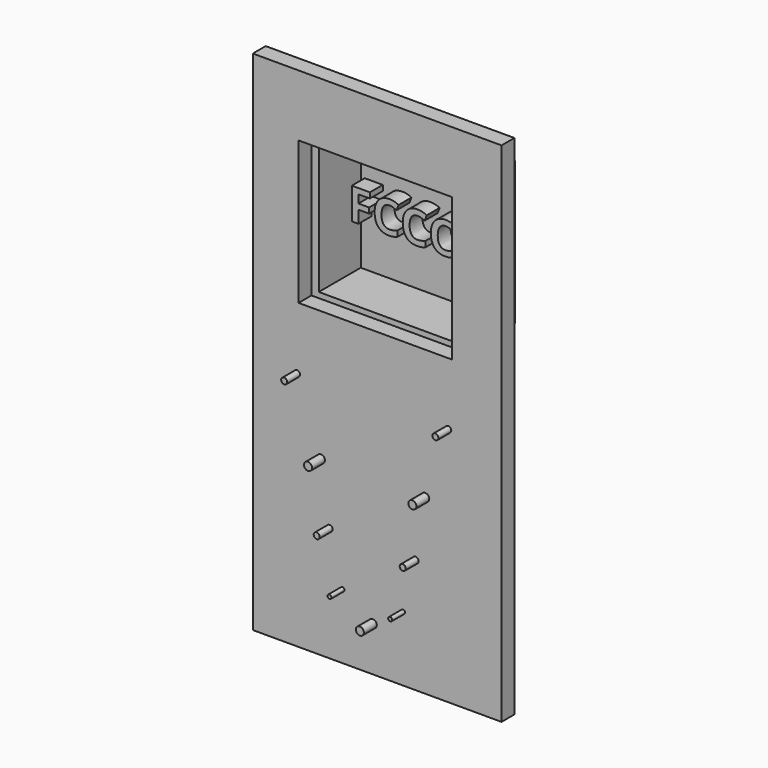
from build123d import *

# Parameters (mm, degrees)
F0_W         = 392.2961652279
F0_H         = 800.5814924836
F0_W_2       = 242.1113476157
F0_H_2       = 225.6477475166
F1_DEPTH     = 25.4
F2_R         = 6.35
F2_R_2       = 3.175
F2_R_3       = 4.7625
F3_DEPTH     = 25.4
F4_W         = 242.1113476157
F4_H         = 225.6477475166
F5_DEPTH     = 99.06
F6_W         = 223.6813679338
F6_H         = 208.9384496212
F7_DEPTH     = 82.804
F8_TEXT_SIZE = 69.5675359498
F9_DEPTH     = 25.4


# Not quite as in the source:
# - Text() gives the source's letters only with a copy of the font that has no kerning and outlines rounded to 1/6400 em; it was checked with that copy


with BuildPart() as f1:
    # F0 (on Front) → F1 (new body)
    with BuildSketch(Plane.XZ):
        with Locations((6.9621950388, 280.5182151496)):
            Rectangle(F0_W, F0_H)
        with Locations((4.0568597615, 470.8177149296)):
            Rectangle(F0_W_2, F0_H_2, mode=Mode.SUBTRACT)
    extrude(amount=F1_DEPTH)

    # F2 (on face) → F3 (join)
    with BuildSketch(Plane.XZ.offset(25.4)):
        with Locations((0, -49.3027232587)):
            Circle(F2_R)
        with Locations((-47.8884726763, -17.2629859298)):
            Circle(F2_R_2)
        with Locations((-68.056344986, 60.8988590539)):
            Circle(F2_R_3)
        with Locations((-81.7621946335, 152.8272628784)):
            Circle(F2_R)
        with Locations((47.8661432862, -17.2629859298)):
            Circle(F2_R_2)
        with Locations((67.6245316863, 60.8988590539)):
            Circle(F2_R_3)
        with Locations((82.7926620841, 152.8272628784)):
            Circle(F2_R)
        with Locations((-119.3668842316, 259.0911984444)):
            Circle(F2_R_3)
        with Locations((119.0826296806, 259.0911984444)):
            Circle(F2_R_3)
    extrude(amount=F3_DEPTH)


with BuildPart() as f5:
    # F4 (on face) → F5 (new body)
    with BuildSketch(Plane(origin=(0, 0, 0), x_dir=(-1, 0, 0), z_dir=(0, 1, 0))):
        with Locations((-4.0568597615, 470.8177149296)):
            Rectangle(F4_W, F4_H)
    extrude(amount=F5_DEPTH)

    # F6 (on face) → F7 (cut)
    with BuildSketch(Plane.XZ):
        with Locations((6.3579715788, 471.0661917925)):
            Rectangle(F6_W, F6_H)
    extrude(amount=-F7_DEPTH, mode=Mode.SUBTRACT)

    # F8 (on face) → F9 (join)
    with BuildSketch(Plane.XZ.offset(-82.804)):
        with Locations((-105.482712388, 443.2695270459)):
            Text('FCCCA', F8_TEXT_SIZE, font='Open Sans', font_style=FontStyle.BOLD, text_align=(TextAlign.LEFT, TextAlign.BOTTOM))
    extrude(amount=F9_DEPTH)


solid = Compound([f1.part, f5.part])
